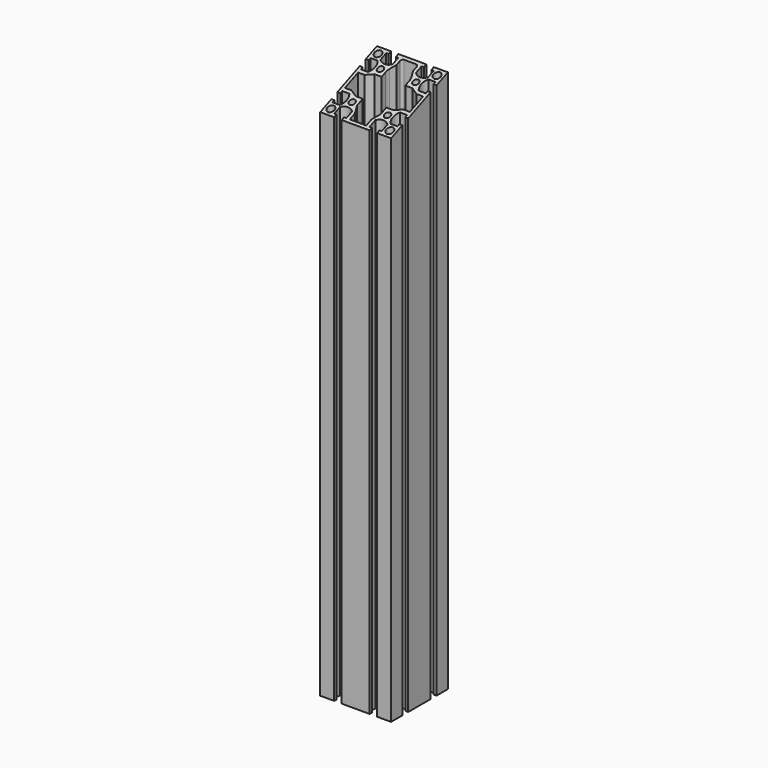
from build123d import *

# Parameters (mm, degrees)
F0_R          = 3
F0_R_2        = 2.5
F1_DEPTH      = 460
F2_R          = 2
F3_R          = 7
F5_DEPTH      = 30
F5_DEPTH_BACK = 30


# Not quite as in the source:
# - a feature names something its author has since deleted; it is built from what else it names


with BuildPart() as f1:
    # F0 (on Top) → F1 (new body)
    with BuildSketch(Plane.XY):
        with BuildLine():
            Line((18.15, -30), (30, -30))
            Line((30, -30), (30, -18.15))
            Line((30, -18.15), (27.5, -18.15))
            Line((27.5, -18.15), (27.5, -20.15))
            Line((27.5, -20.15), (21.5477069044, -20.15))
            ThreePointArc((21.5477069044, -20.15), (19.5, -15), (21.5477069044, -9.85))
            Line((21.5477069044, -9.85), (27.5, -9.85))
            Line((27.5, -9.85), (27.5, -11.85))
            Line((27.5, -11.85), (30, -11.85))
            Line((30, -11.85), (30, 11.85))
            Line((30, 11.85), (27.5, 11.85))
            Line((27.5, 11.85), (27.5, 9.85))
            Line((27.5, 9.85), (21.5477069044, 9.85))
            ThreePointArc((21.5477069044, 9.85), (19.5, 15), (21.5477069044, 20.15))
            Line((21.5477069044, 20.15), (27.5, 20.15))
            Line((27.5, 20.15), (27.5, 18.15))
            Line((27.5, 18.15), (30, 18.15))
            Line((30, 18.15), (30, 30))
            Line((30, 30), (18.15, 30))
            Line((18.15, 30), (18.15, 27.5))
            Line((18.15, 27.5), (20.15, 27.5))
            Line((20.15, 27.5), (20.15, 21.5477069044))
            ThreePointArc((20.15, 21.5477069044), (15, 19.5), (9.85, 21.5477069044))
            Line((9.85, 21.5477069044), (9.85, 27.5))
            Line((9.85, 27.5), (11.85, 27.5))
            Line((11.85, 27.5), (11.85, 30))
            Line((11.85, 30), (-11.85, 30))
            Line((-11.85, 30), (-11.85, 27.5))
            Line((-11.85, 27.5), (-9.85, 27.5))
            Line((-9.85, 27.5), (-9.85, 21.5477069044))
            ThreePointArc((-9.85, 21.5477069044), (-15, 19.5), (-20.15, 21.5477069044))
            Line((-20.15, 21.5477069044), (-20.15, 27.5))
            Line((-20.15, 27.5), (-18.15, 27.5))
            Line((-18.15, 27.5), (-18.15, 30))
            Line((-18.15, 30), (-30, 30))
            Line((-30, 30), (-30, 18.15))
            Line((-30, 18.15), (-27.5, 18.15))
            Line((-27.5, 18.15), (-27.5, 20.15))
            Line((-27.5, 20.15), (-21.5477069044, 20.15))
            ThreePointArc((-21.5477069044, 20.15), (-19.5, 15), (-21.5477069044, 9.85))
            Line((-21.5477069044, 9.85), (-27.5, 9.85))
            Line((-27.5, 9.85), (-27.5, 11.85))
            Line((-27.5, 11.85), (-30, 11.85))
            Line((-30, 11.85), (-30, -11.85))
            Line((-30, -11.85), (-27.5, -11.85))
            Line((-27.5, -11.85), (-27.5, -9.85))
            Line((-27.5, -9.85), (-21.5477069044, -9.85))
            ThreePointArc((-21.5477069044, -9.85), (-19.5, -15), (-21.5477069044, -20.15))
            Line((-21.5477069044, -20.15), (-27.5, -20.15))
            Line((-27.5, -20.15), (-27.5, -18.15))
            Line((-27.5, -18.15), (-30, -18.15))
            Line((-30, -18.15), (-30, -30))
            Line((-30, -30), (-18.15, -30))
            Line((-18.15, -30), (-18.15, -27.5))
            Line((-18.15, -27.5), (-20.15, -27.5))
            Line((-20.15, -27.5), (-20.15, -21.5477069044))
            ThreePointArc((-20.15, -21.5477069044), (-15, -19.5), (-9.85, -21.5477069044))
            Line((-9.85, -21.5477069044), (-9.85, -27.5))
            Line((-9.85, -27.5), (-11.85, -27.5))
            Line((-11.85, -27.5), (-11.85, -30))
            Line((-11.85, -30), (11.85, -30))
            Line((11.85, -30), (11.85, -27.5))
            Line((11.85, -27.5), (9.85, -27.5))
            Line((9.85, -27.5), (9.85, -21.5477069044))
            ThreePointArc((9.85, -21.5477069044), (15, -19.5), (20.15, -21.5477069044))
            Line((20.15, -21.5477069044), (20.15, -27.5))
            Line((20.15, -27.5), (18.15, -27.5))
            Line((18.15, -27.5), (18.15, -30))
        make_face()
        with Locations((-25, -25)):
            Circle(F0_R, mode=Mode.SUBTRACT)
        with Locations((-15, -15)):
            Circle(F0_R_2, mode=Mode.SUBTRACT)
        with Locations((25, -25)):
            Circle(F0_R, mode=Mode.SUBTRACT)
        with Locations((15, -15)):
            Circle(F0_R_2, mode=Mode.SUBTRACT)
        with Locations((-25, 25)):
            Circle(F0_R, mode=Mode.SUBTRACT)
        with Locations((-15, 15)):
            Circle(F0_R_2, mode=Mode.SUBTRACT)
        Polygon((-7, 22), (-7, 27.5), (0, 27.5), (7, 27.5), (7, 22), (10, 16), (10, 10), (16, 10), (22, 7), (27.5, 7), (27.5, 0), (27.5, -7), (22, -7), (16, -10), (10, -10), (10, -16), (7, -22), (7, -27.5), (0, -27.5), (-7, -27.5), (-7, -22), (-10, -16), (-10, -10), (-16, -10), (-22, -7), (-27.5, -7), (-27.5, 0), (-27.5, 7), (-22, 7), (-16, 10), (-10, 10), (-10, 16), align=None, mode=Mode.SUBTRACT)
        with Locations((15, 15)):
            Circle(F0_R_2, mode=Mode.SUBTRACT)
        with Locations((25, 25)):
            Circle(F0_R, mode=Mode.SUBTRACT)
    extrude(amount=F1_DEPTH)

    # F2
    f2_edges = [f1.edges().sort_by_distance(p)[0] for p in [
        (-7, 27.5, 230),
        (7, 27.5, 230),
    ]]
    fillet(f2_edges, radius=F2_R)

    # F3
    f3_edges = [f1.edges().sort_by_distance(p)[0] for p in [
        (-10, 16, 230),
        (10, 16, 230),
    ]]
    fillet(f3_edges, radius=F3_R)

    # F4 (on Right) → F5 (cut, two sides)
    with BuildSketch(Plane.YZ) as f5_sk:
        Polygon((30, 460), (-101.7983138763, 778.1892768581), (-315.3200388241, 689.7456825234), (-183.5217249478, 371.5564056653), align=None)
    extrude(amount=F5_DEPTH, mode=Mode.SUBTRACT)
    extrude(f5_sk.sketch, amount=-F5_DEPTH_BACK, mode=Mode.SUBTRACT)


solid = f1.part
